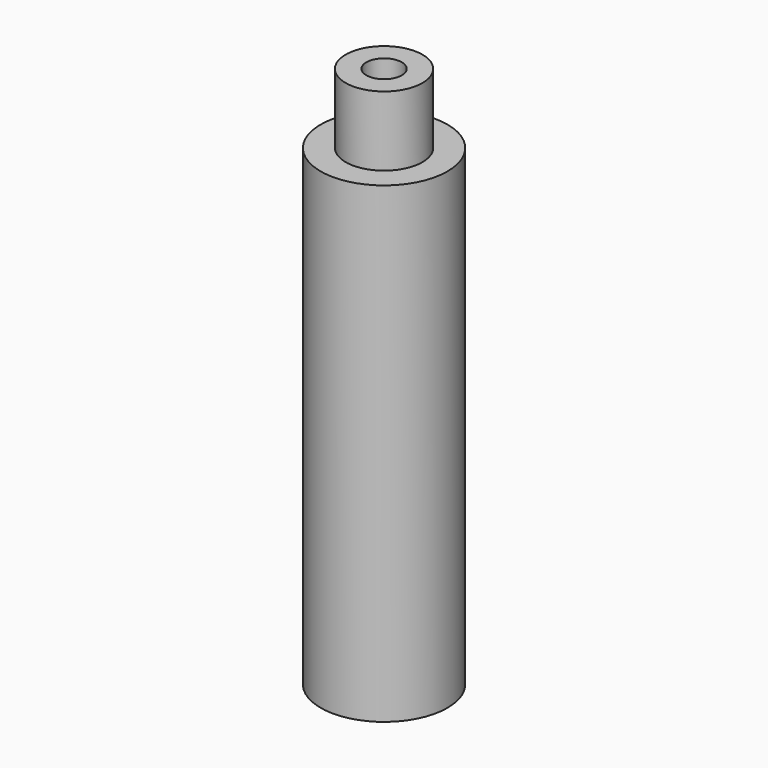
from build123d import *

# Parameters (mm, degrees)
F0_R     = 3.7338
F1_DEPTH = 27.8003
F2_R     = 2.2606
F3_DEPTH = 4.1021
F4_R     = 1.0414
F5_DEPTH = 47.0154
F6_R     = 2.53873
F7_DEPTH = 26.9494
F8_R     = 3.7338
F9_DEPTH = 26.3144


with BuildPart() as f1:
    # F0 (on Top) → F1 (new body)
    with BuildSketch(Plane.XY):
        Circle(F0_R)
    extrude(amount=F1_DEPTH)

    # F2 (on face) → F3 (join)
    with BuildSketch(Plane.XY.offset(27.8003)):
        Circle(F2_R)
    extrude(amount=F3_DEPTH)

    # F4 (on face) → F5 (cut)
    with BuildSketch(Plane.XY.offset(31.9024)):
        Circle(F4_R)
    extrude(amount=-F5_DEPTH, mode=Mode.SUBTRACT)

    # F6 (on face) → F7 (cut)
    with BuildSketch(Plane(origin=(0, 0, 0), x_dir=(1, 0, 0), z_dir=(0, 0, -1))):
        Circle(F6_R)
    extrude(amount=-F7_DEPTH, mode=Mode.SUBTRACT)

    # F8 (on face) → F9 (join)
    with BuildSketch(Plane(origin=(0, 0, 0), x_dir=(1, 0, 0), z_dir=(0, 0, -1))):
        Circle(F8_R)
        with BuildLine():
            Line((1.1798710111, 2.2479), (2.2479, 2.2479))
            Line((2.2479, 2.2479), (2.2479, 1.1798710111))
            ThreePointArc((2.2479, 1.1798710111), (2.4649504234, 0.6075931393), (2.53873, 0))
            ThreePointArc((2.53873, 0), (2.4649504234, -0.6075931393), (2.2479, -1.1798710111))
            Line((2.2479, -1.1798710111), (2.2479, -2.2479))
            Line((2.2479, -2.2479), (1.1798710111, -2.2479))
            ThreePointArc((1.1798710111, -2.2479), (0, -2.53873), (-1.1798710111, -2.2479))
            Line((-1.1798710111, -2.2479), (-2.2479, -2.2479))
            Line((-2.2479, -2.2479), (-2.2479, -1.1798710111))
            ThreePointArc((-2.2479, -1.1798710111), (-2.53873, 0), (-2.2479, 1.1798710111))
            Line((-2.2479, 1.1798710111), (-2.2479, 2.2479))
            Line((-2.2479, 2.2479), (-1.1798710111, 2.2479))
            ThreePointArc((-1.1798710111, 2.2479), (0, 2.53873), (1.1798710111, 2.2479))
        make_face(mode=Mode.SUBTRACT)
        with BuildLine():
            Line((-1.1798710111, 2.2479), (1.1798710111, 2.2479))
            ThreePointArc((1.1798710111, 2.2479), (0, 2.53873), (-1.1798710111, 2.2479))
        make_face()
        with BuildLine():
            ThreePointArc((2.53873, 0), (2.4649504234, 0.6075931393), (2.2479, 1.1798710111))
            Line((2.2479, 1.1798710111), (2.2479, -1.1798710111))
            ThreePointArc((2.2479, -1.1798710111), (2.4649504234, -0.6075931393), (2.53873, 0))
        make_face()
        with BuildLine():
            Line((-2.2479, -1.1798710111), (-2.2479, 1.1798710111))
            ThreePointArc((-2.2479, 1.1798710111), (-2.53873, 0), (-2.2479, -1.1798710111))
        make_face()
        with BuildLine():
            ThreePointArc((-1.1798710111, -2.2479), (0, -2.53873), (1.1798710111, -2.2479))
            Line((1.1798710111, -2.2479), (-1.1798710111, -2.2479))
        make_face()
    extrude(amount=-F9_DEPTH)


solid = f1.part
